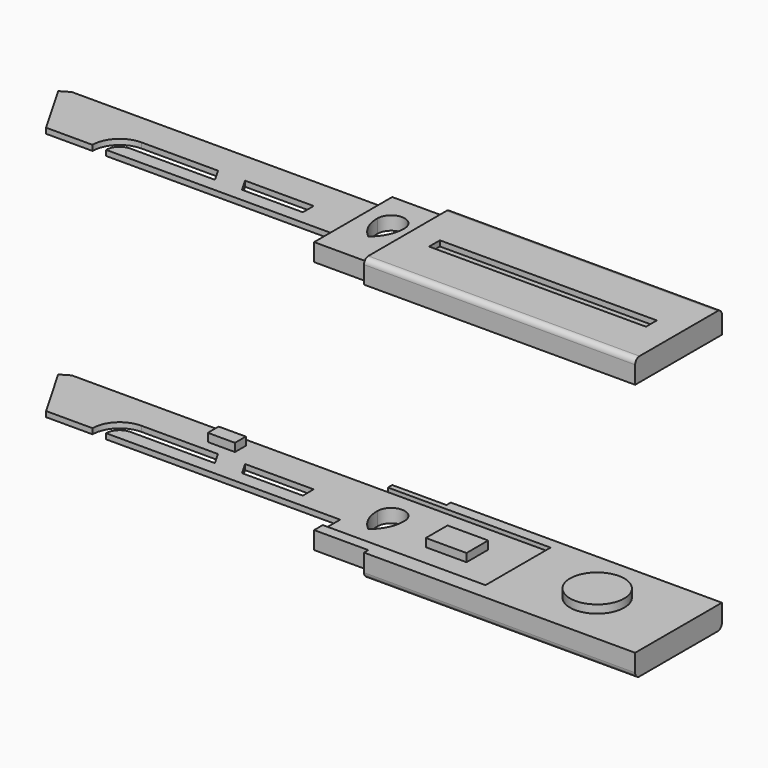
from build123d import *

# Parameters (mm, degrees)
F0_W      = 20
F0_H      = 36
F1_DEPTH  = 6.5
F3_W      = 22
F3_H      = 3.5
F4_DEPTH  = 120
F2_W      = 30
F2_H      = 1.5
F5_DEPTH  = 140.001
F7_DEPTH  = 25
F8_W      = 40
F8_H      = 8.5
F9_DEPTH  = 100
F10_DEPTH = 40
F13_W     = 10
F13_H     = 5
F13_W_2   = 15
F13_H_2   = 10
F14_DEPTH = 3
F16_DEPTH = 102.001
F17_W     = 80
F17_H     = 5
F18_DEPTH = 2
F21_W     = 80
F21_H     = 5
F22_DEPTH = 2
F25_R     = 2
F25_2_R   = 2
F27_R     = 10
F28_DEPTH = 3
F26_R     = 10
F29_DEPTH = 3


# Not quite as in the source:
# - the program builds the solid bodies; features that only make, move or delete a surface that nothing else refers to are left out


with BuildPart() as f1:
    # F0 (on Top) → F1 (new body)
    with BuildSketch(Plane.XY):
        with Locations((-13.2614625618, -0.0489673983)):
            Rectangle(F0_W, F0_H)
    extrude(amount=F1_DEPTH)

    # F3 (on face) → F4 (join)
    with BuildSketch(Plane(origin=(-23.2614625618, 0, 0), x_dir=(0, -1, 0), z_dir=(-1, 0, 0))):
        with Locations((-4.9510326017, 4.75)):
            Rectangle(F3_W, F3_H)
    extrude(amount=F4_DEPTH)

    # F2 (on face) → F5 (cut, through all)
    with BuildSketch(Plane.YZ.offset(-3.2614625618)):
        with Locations((0.9510326017, 5.75)):
            Rectangle(F2_W, F2_H)
    extrude(amount=-F5_DEPTH, mode=Mode.SUBTRACT)

    # F6 (on face) → F7 (cut)
    with BuildSketch(Plane(origin=(0, 0, 3), x_dir=(1, 0, 0), z_dir=(0, 0, -1))):
        Polygon((-41.026044637, 1.0489673983), (-63.4366088587, 1.0489673983), (-66.3233602047, -3.9510326017), (-41.026044637, -3.9510326017), align=None)
        Polygon((-143.2614625618, 6.0489673983), (-143.2614625618, -13.9510326017), (-131.714457178, 6.0489673983), align=None)
        Polygon((-139.7973609466, -15.9510326017), (-143.2614625618, -13.9510326017), (-143.2614625618, -15.9510326017), align=None)
        with BuildLine():
            Line((-109.5855507255, 6.0489673983), (-114.5855507255, 6.0489673983))
            ThreePointArc((-114.5855507255, 6.0489673983), (-111.6566185373, -1.0221004135), (-104.5855507255, -3.9510326017))
            Line((-104.5855507255, -3.9510326017), (-76.3233602047, -3.9510326017))
            Line((-76.3233602047, -3.9510326017), (-73.4366088587, 1.0489673983))
            Line((-73.4366088587, 1.0489673983), (-104.5855507255, 1.0489673983))
            ThreePointArc((-104.5855507255, 1.0489673983), (-108.1210846314, 2.5134334924), (-109.5855507255, 6.0489673983))
        make_face()
    extrude(amount=-F7_DEPTH, mode=Mode.SUBTRACT)

    # F8 (on face) → F9 (join)
    with BuildSketch(Plane.YZ.offset(-3.2614625618)):
        with Locations((-0.0489673983, 2.25)):
            Rectangle(F8_W, F8_H)
    extrude(amount=F9_DEPTH)

    # F10 (cut): a face of the model
    f10_faces = [f1.faces().sort_by_distance(p)[0] for p in [
        (-3.2614625618, 0.9510326017, 5.75),
    ]]
    extrude(f10_faces, amount=-F10_DEPTH, mode=Mode.SUBTRACT)


with BuildPart() as f12_1:
    # F12: instance of F1
    add(f1.part.mirror(Plane.XY.offset(50)))


with BuildPart() as f1_1:
    add(f1.part)

    # F13 (on face) → F14 (join)
    with BuildSketch(Plane.XY.offset(5)):
        with Locations((-78.2614625618, 10.4510326017)):
            Rectangle(F13_W, F13_H)
        with Locations((14.2385374382, 0.9510326017)):
            Rectangle(F13_W_2, F13_H_2)
    extrude(amount=F14_DEPTH)


with BuildPart() as f16_tool:
    # F15 (on face) → F16 (new body, through all)
    with BuildSketch(Plane.XY):
        with BuildLine():
            ThreePointArc((-18.2614625618, 4.9510326017), (-13.2614625618, -0.0489673983), (-8.2614625618, 4.9510326017))
            ThreePointArc((-8.2614625618, 4.9510326017), (-13.2614625618, 9.9510326017), (-18.2614625618, 4.9510326017))
        make_face()
        with BuildLine():
            ThreePointArc((-13.2614625618, -5.5633480661), (-9.5186017181, -0.8971867633), (-8.2614625618, 4.9510326017))
            ThreePointArc((-8.2614625618, 4.9510326017), (-13.2614625618, -0.0489673983), (-18.2614625618, 4.9510326017))
            ThreePointArc((-18.2614625618, 4.9510326017), (-17.0043234055, -0.8971867633), (-13.2614625618, -5.5633480661))
        make_face()
    extrude(amount=F16_DEPTH)


with BuildPart() as f1_2:
    add(f1_1.part)

    # F16: cut by f16_tool
    add(f16_tool.part, mode=Mode.SUBTRACT)

    # F17 (on face) → F18 (cut)
    with BuildSketch(Plane(origin=(0, 0, -2), x_dir=(1, 0, 0), z_dir=(0, 0, -1))):
        with Locations((46.7385374382, 0.0489673983)):
            Rectangle(F17_W, F17_H)
    extrude(amount=-F18_DEPTH, mode=Mode.SUBTRACT)

    # F25
    f25_edges = [f1_2.edges().sort_by_distance(p)[0] for p in [
        (46.738537, 19.951033, -2),
        (46.738537, -20.048967, -2),
    ]]
    fillet(f25_edges, radius=F25_R)

    # F26 (on face) → F29 (join)
    with BuildSketch(Plane.XY.offset(6.5)):
        with Locations((66.7385374382, -0.0489673983)):
            Circle(F26_R)
    extrude(amount=F29_DEPTH)


with BuildPart() as f12_1_1:
    add(f12_1.part)

    # F16: cut by f16_tool
    add(f16_tool.part, mode=Mode.SUBTRACT)

    # F21 (on face) → F22 (cut)
    with BuildSketch(Plane.XY.offset(102)):
        with Locations((46.7385374382, -0.0489673983)):
            Rectangle(F21_W, F21_H)
    extrude(amount=-F22_DEPTH, mode=Mode.SUBTRACT)

    # F25#2
    f25_2_edges = [f12_1_1.edges().sort_by_distance(p)[0] for p in [
        (46.738537, -20.048967, 102),
        (46.738537, 19.951033, 102),
    ]]
    fillet(f25_2_edges, radius=F25_2_R)

    # F27 (on face) → F28 (cut)
    with BuildSketch(Plane(origin=(0, 0, 93.5), x_dir=(1, 0, 0), z_dir=(0, 0, -1))):
        with Locations((66.7385374382, 0.0489673983)):
            Circle(F27_R)
    extrude(amount=-F28_DEPTH, mode=Mode.SUBTRACT)


solid = Compound([f1_2.part, f12_1_1.part])
